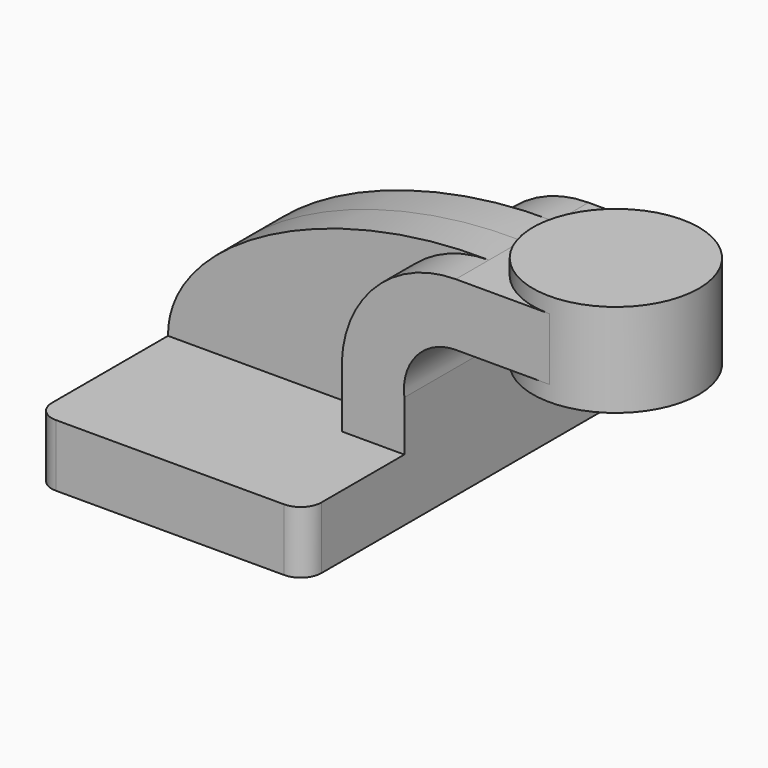
from build123d import *

# Parameters (mm, degrees)
F1_DEPTH = 63.5
F0_W     = 25.4
F0_H     = 19.05
F2_DEPTH = 25.4
F3_DEPTH = 12.7
F5_R     = 6.35


# Not quite as in the source:
# - a feature names something its author has since deleted; it is built from what else it names


with BuildPart() as f1:
    # F0 (on Front) → F1 (new body, symmetric)
    with BuildSketch(Plane.XZ):
        Polygon((-41.275, 9.525), (-41.275, -9.525), (41.275, -9.525), (41.275, 9.525), (22.225, 9.525), align=None)
    extrude(amount=F1_DEPTH, both=True)

    # F0 (on Front) → F2 (join, symmetric)
    with BuildSketch(Plane.XZ):
        with BuildLine():
            Line((22.225, 9.525), (41.275, 9.525))
            Line((41.275, 9.525), (41.275, 24.9272808433))
            ThreePointArc((41.275, 24.9272808433), (45.0783515165, 37.4670054674), (57.0140797434, 42.8752))
            Line((57.0140797434, 42.8752), (60.325, 42.8752))
            Line((60.325, 42.8752), (60.325, 61.9252))
            Line((60.325, 61.9252), (57.0140797434, 61.9252))
            ThreePointArc((57.0140797434, 61.9252), (31.2530323697, 50.5824828244), (22.225, 23.9219609569))
            Line((22.225, 23.9219609569), (22.225, 9.525))
        make_face()
        with Locations((73.025, 52.4002)):
            Rectangle(F0_W, F0_H)
    extrude(amount=F2_DEPTH, both=True)

    # F0 (on Front) → F3 (join, symmetric)
    with BuildSketch(Plane.XZ):
        with BuildLine():
            add(Edge.make_bspline(
                [(57.0140797434, 61.9252), (7.5895511545, 62.9258826375), (-41.465934366, 37.4339222908), (-41.275, 9.525)],
                knots=[0, 0, 0, 0, 111.3845777334, 111.3845777334, 111.3845777334, 111.3845777334], degree=3))
            Line((-41.275, 9.525), (22.225, 9.525))
            Line((22.225, 9.525), (22.225, 23.9219609569))
            ThreePointArc((22.225, 23.9219609569), (31.2530323697, 50.5824828244), (57.0140797434, 61.9252))
        make_face()
    extrude(amount=F3_DEPTH, both=True)

    # F5
    f5_edges = [f1.edges().sort_by_distance(p)[0] for p in [
        (41.275, -63.5, 0),
        (-41.275, -63.5, 0),
        (-41.275, 63.5, 0),
        (41.275, 63.5, 0),
    ]]
    fillet(f5_edges, radius=F5_R)


with BuildPart() as f4:
    # F0 (on Front) → F4 (revolve)
    with BuildSketch(Plane.XZ):
        Polygon((85.725, 66.675), (85.725, 61.9252), (85.725, 42.8752), (85.725, 38.1), (111.125, 38.1), (111.125, 66.675), align=None)
    revolve(axis=Axis((85.725, 0, 52.3875), (0, 0, 1)))


solid = Compound([f1.part, f4.part])
